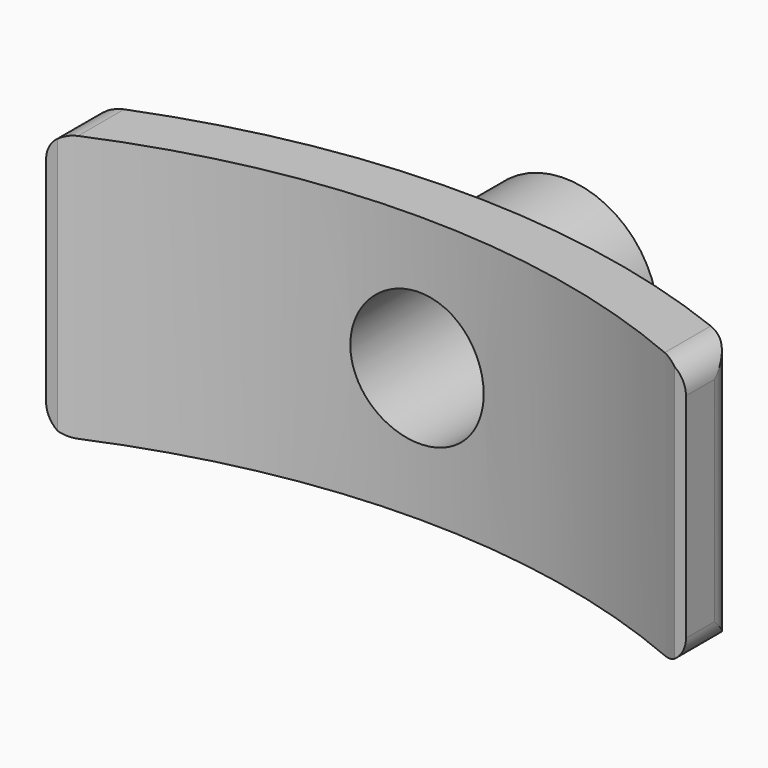
from build123d import *

# Parameters (mm, degrees)
F1_DEPTH = 50
F3_START = -144.7303891182
F2_R     = 17.5
F3_DEPTH = 29.2989462614
F4_R     = 5
F6_D     = 25
F7_R     = 5


with BuildPart() as f1:
    # F0 (on Top) → F1 (new body)
    with BuildSketch(Plane.XY):
        with BuildLine():
            ThreePointArc((-57.8447732054, 127.4911064067), (0, 140), (57.8447732054, 127.4911064067))
            Line((57.8447732054, 127.4911064067), (60, 127.4911064067))
            Line((60, 127.4911064067), (60, 137.4772708487))
            ThreePointArc((60, 137.4772708487), (0, 150), (-60, 137.4772708487))
            Line((-60, 137.4772708487), (-60, 127.4911064067))
            Line((-60, 127.4911064067), (-57.8447732054, 127.4911064067))
        make_face()
    extrude(amount=F1_DEPTH)

    # F2 (on Front) → F3 (join)
    with BuildSketch(Plane.XZ.offset(F3_START)):
        with Locations((0, 25)):
            Circle(F2_R)
    extrude(amount=-F3_DEPTH)

    # F4
    f4_edges = [f1.edges().sort_by_distance(p)[0] for p in [
        (-17.5, 148.975669, 25),
    ]]
    fillet(f4_edges, radius=F4_R)

    # F6 (through all)
    with Locations(Plane(origin=(0, 174.0293353796, 0), x_dir=(-1, 0, 0), z_dir=(0, 1, 0))):
        with Locations((0, 25)):
            Hole(F6_D / 2)

    # F7
    f7_edges = [f1.edges().sort_by_distance(p)[0] for p in [
        (-60, 132.484189, 50),
        (-60, 137.477271, 25),
        (-60, 132.484189, 0),
        (60, 132.484189, 50),
        (60, 137.477271, 25),
        (60, 132.484189, 0),
    ]]
    fillet(f7_edges, radius=F7_R)


solid = f1.part
